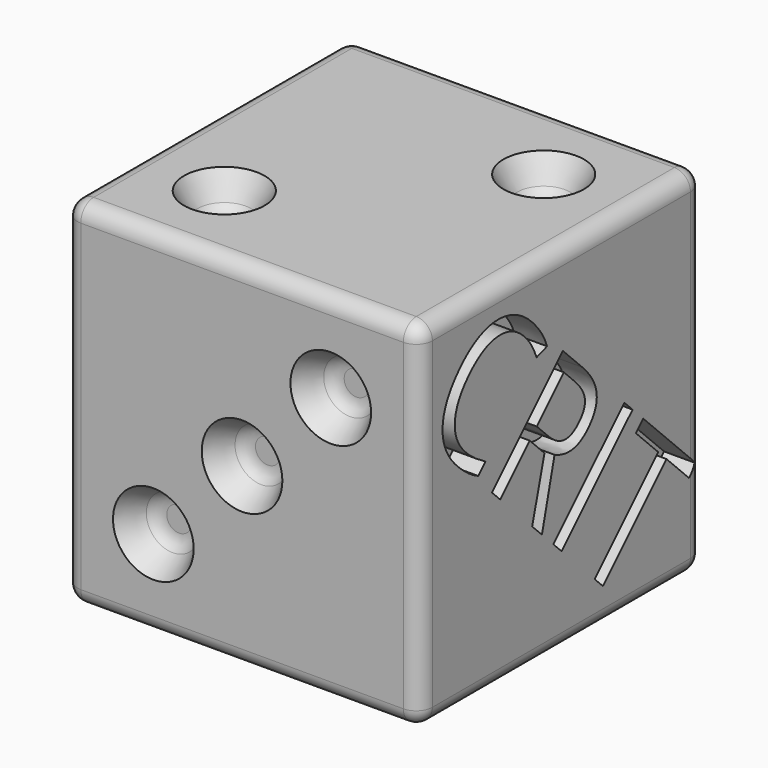
from build123d import *

# Parameters (mm, degrees)
F0_W          = 22
F0_H          = 22
F1_DEPTH      = 22
F2_R          = 2.5
F3_DEPTH      = 2
F3_TAPER      = 30
F4_R          = 2.5
F5_DEPTH      = 2
F5_TAPER      = 30
F6_R          = 2.5
F7_DEPTH      = 2
F7_TAPER      = 30
F8_R          = 2.5
F9_DEPTH      = 2
F9_TAPER      = 30
F10_R         = 2.5
F11_DEPTH     = 2
F11_TAPER     = 30
F12_TEXT_SIZE = 10.8916567981
F13_DEPTH     = 2
F14_T31_DEPTH = 20
F14_T33_DEPTH = 20
F14_T35_DEPTH = 20
F14_S39_W     = 1
F14_S39_H     = 1
F14_T40_DEPTH = 1
F14_S45_W     = 1
F14_S45_H     = 1
F14_T46_DEPTH = 1
F14_S51_W     = 1
F14_S51_H     = 1
F14_T52_DEPTH = 1
F14_S57_W     = 1
F14_S57_H     = 1
F14_T58_DEPTH = 1
F14_S63_W     = 1
F14_S63_H     = 1
F14_T64_DEPTH = 1
F14_S69_W     = 1
F14_S69_H     = 1
F14_T70_DEPTH = 1
F14_S75_W     = 1
F14_S75_H     = 1
F14_T76_DEPTH = 1
F14_S81_W     = 1
F14_S81_H     = 1
F14_T82_DEPTH = 1


# Not quite as in the source:
# - a fillet or chamfer that OpenCascade refuses, or shapes differently, is made with other operations: its cross-section is extruded or revolved along the edge and cut away or added
# - Text() gives the source's letters only with a copy of the font that has no kerning and outlines rounded to 1/6400 em; it was checked with that copy


with BuildPart() as f1:
    # F0 (on Top) → F1 (new body)
    with BuildSketch(Plane.XY):
        Rectangle(F0_W, F0_H)
    extrude(amount=F1_DEPTH)

    # F2 (on face) → F3 (cut)
    with BuildSketch(Plane(origin=(-11, 0, 0), x_dir=(0, -1, 0), z_dir=(-1, 0, 0))):
        with Locations((0, 11)):
            Circle(F2_R)
    extrude(amount=-F3_DEPTH, taper=F3_TAPER, mode=Mode.SUBTRACT)

    # F4 (on face) → F5 (cut)
    with BuildSketch(Plane.XY.offset(22)):
        with Locations((5.5, 5.5)):
            Circle(F4_R)
        with Locations((-5.5, -5.5)):
            Circle(F4_R)
    extrude(amount=-F5_DEPTH, taper=F5_TAPER, mode=Mode.SUBTRACT)

    # F6 (on face) → F7 (cut)
    with BuildSketch(Plane.XZ.offset(11)):
        with Locations((5.5, 16.5)):
            Circle(F6_R)
        with Locations((0, 11)):
            Circle(F6_R)
        with Locations((-5.5, 5.5)):
            Circle(F6_R)
    extrude(amount=-F7_DEPTH, taper=F7_TAPER, mode=Mode.SUBTRACT)

    # F8 (on face) → F9 (cut)
    with BuildSketch(Plane(origin=(0, 11, 0), x_dir=(-1, 0, 0), z_dir=(0, 1, 0))):
        with Locations((5.5, 16.5)):
            Circle(F8_R)
        with Locations((-5.5, 16.5)):
            Circle(F8_R)
        with Locations((5.5, 5.5)):
            Circle(F8_R)
        with Locations((-5.5, 5.5)):
            Circle(F8_R)
    extrude(amount=-F9_DEPTH, taper=F9_TAPER, mode=Mode.SUBTRACT)

    # F10 (on face) → F11 (cut)
    with BuildSketch(Plane(origin=(0, 0, 0), x_dir=(1, 0, 0), z_dir=(0, 0, -1))):
        Circle(F10_R)
        with Locations((5.5, -5.5)):
            Circle(F10_R)
        with Locations((-5.5, 5.5)):
            Circle(F10_R)
        with Locations((5.5, 5.5)):
            Circle(F10_R)
        with Locations((-5.5, -5.5)):
            Circle(F10_R)
    extrude(amount=-F11_DEPTH, taper=F11_TAPER, mode=Mode.SUBTRACT)

    # F12 (on face) → F13 (cut)
    with BuildSketch(Plane.YZ.offset(11)):
        with Locations(Location((-11, 16.4548736462), (0, 0, -45))):
            Text('CRIT', F12_TEXT_SIZE, font='Open Sans', text_align=(TextAlign.LEFT, TextAlign.BOTTOM))
    extrude(amount=-F13_DEPTH, mode=Mode.SUBTRACT)

    # F14: fillet of radius 1 on 27 edges, made by hand

    # F14_s1 → F14_t2 (revolve)
    with BuildSketch(Plane.XY.offset(16.5)):
        with BuildLine():
            ThreePointArc((-7.1339745962, 9.5), (-6.7679491924, 9.1339745962), (-6.2679491924, 9))
            Line((-6.2679491924, 9), (-6.8452994616, 9))
            Line((-6.8452994616, 9), (-7.1339745962, 9.5))
        make_face()
    revolve(axis=Axis((-5.5, 9, 16.5), (0, 1, 0)))

    # F14_s3 → F14_t4 (revolve)
    with BuildSketch(Plane.XY.offset(5.5)):
        with BuildLine():
            ThreePointArc((-7.1339745962, 9.5), (-6.7679491924, 9.1339745962), (-6.2679491924, 9))
            Line((-6.2679491924, 9), (-6.8452994616, 9))
            Line((-6.8452994616, 9), (-7.1339745962, 9.5))
        make_face()
    revolve(axis=Axis((-5.5, 9, 5.5), (0, 1, 0)))

    # F14_s5 → F14_t6 (revolve)
    with BuildSketch(Plane.XY.offset(5.5)):
        with BuildLine():
            ThreePointArc((3.8660254038, 9.5), (4.2320508076, 9.1339745962), (4.7320508076, 9))
            Line((4.7320508076, 9), (4.1547005384, 9))
            Line((4.1547005384, 9), (3.8660254038, 9.5))
        make_face()
    revolve(axis=Axis((5.5, 9, 5.5), (0, 1, 0)))

    # F14_s7 → F14_t8 (revolve)
    with BuildSketch(Plane.XY.offset(16.5)):
        with BuildLine():
            ThreePointArc((3.8660254038, 9.5), (4.2320508076, 9.1339745962), (4.7320508076, 9))
            Line((4.7320508076, 9), (4.1547005384, 9))
            Line((4.1547005384, 9), (3.8660254038, 9.5))
        make_face()
    revolve(axis=Axis((5.5, 9, 16.5), (0, 1, 0)))

    # F14_s9 → F14_t10 (revolve)
    with BuildSketch(Plane.XZ.offset(-5.5)):
        with BuildLine():
            ThreePointArc((7.1339745962, 20.5), (6.7679491924, 20.1339745962), (6.2679491924, 20))
            Line((6.2679491924, 20), (6.8452994616, 20))
            Line((6.8452994616, 20), (7.1339745962, 20.5))
        make_face()
    revolve(axis=Axis((5.5, 5.5, 20), (0, 0, 1)))

    # F14_s11 → F14_t12 (revolve)
    with BuildSketch(Plane.XZ.offset(5.5)):
        with BuildLine():
            ThreePointArc((-3.8660254038, 20.5), (-4.2320508076, 20.1339745962), (-4.7320508076, 20))
            Line((-4.7320508076, 20), (-4.1547005384, 20))
            Line((-4.1547005384, 20), (-3.8660254038, 20.5))
        make_face()
    revolve(axis=Axis((-5.5, -5.5, 20), (0, 0, 1)))

    # F14_s13 → F14_t14 (revolve)
    with BuildSketch(Plane.XZ.offset(-5.5)):
        with BuildLine():
            ThreePointArc((-3.8660254038, 1.5), (-4.2320508076, 1.8660254038), (-4.7320508076, 2))
            Line((-4.7320508076, 2), (-4.1547005384, 2))
            Line((-4.1547005384, 2), (-3.8660254038, 1.5))
        make_face()
    revolve(axis=Axis((-5.5, 5.5, 2), (0, 0, -1)))

    # F14_s15 → F14_t16 (revolve)
    with BuildSketch(Plane.XZ.offset(-5.5)):
        with BuildLine():
            ThreePointArc((7.1339745962, 1.5), (6.7679491924, 1.8660254038), (6.2679491924, 2))
            Line((6.2679491924, 2), (6.8452994616, 2))
            Line((6.8452994616, 2), (7.1339745962, 1.5))
        make_face()
    revolve(axis=Axis((5.5, 5.5, 2), (0, 0, -1)))

    # F14_s17 → F14_t18 (revolve)
    with BuildSketch(Plane.XZ):
        with BuildLine():
            ThreePointArc((1.6339745962, 1.5), (1.2679491924, 1.8660254038), (0.7679491924, 2))
            Line((0.7679491924, 2), (1.3452994616, 2))
            Line((1.3452994616, 2), (1.6339745962, 1.5))
        make_face()
    revolve(axis=Axis((0, 0, 2), (0, 0, -1)))

    # F14_s19 → F14_t20 (revolve)
    with BuildSketch(Plane.XZ.offset(5.5)):
        with BuildLine():
            ThreePointArc((7.1339745962, 1.5), (6.7679491924, 1.8660254038), (6.2679491924, 2))
            Line((6.2679491924, 2), (6.8452994616, 2))
            Line((6.8452994616, 2), (7.1339745962, 1.5))
        make_face()
    revolve(axis=Axis((5.5, -5.5, 2), (0, 0, -1)))

    # F14_s21 → F14_t22 (revolve)
    with BuildSketch(Plane.XZ.offset(5.5)):
        with BuildLine():
            ThreePointArc((-3.8660254038, 1.5), (-4.2320508076, 1.8660254038), (-4.7320508076, 2))
            Line((-4.7320508076, 2), (-4.1547005384, 2))
            Line((-4.1547005384, 2), (-3.8660254038, 1.5))
        make_face()
    revolve(axis=Axis((-5.5, -5.5, 2), (0, 0, -1)))

    # F14_s23 → F14_t24 (revolve)
    with BuildSketch(Plane.XY.offset(5.5)):
        with BuildLine():
            ThreePointArc((-3.8660254038, -9.5), (-4.2320508076, -9.1339745962), (-4.7320508076, -9))
            Line((-4.7320508076, -9), (-4.1547005384, -9))
            Line((-4.1547005384, -9), (-3.8660254038, -9.5))
        make_face()
    revolve(axis=Axis((-5.5, -9, 5.5), (0, -1, 0)))

    # F14_s25 → F14_t26 (revolve)
    with BuildSketch(Plane.XY.offset(11)):
        with BuildLine():
            ThreePointArc((1.6339745962, -9.5), (1.2679491924, -9.1339745962), (0.7679491924, -9))
            Line((0.7679491924, -9), (1.3452994616, -9))
            Line((1.3452994616, -9), (1.6339745962, -9.5))
        make_face()
    revolve(axis=Axis((0, -9, 11), (0, -1, 0)))

    # F14_s27 → F14_t28 (revolve)
    with BuildSketch(Plane.XY.offset(11)):
        with BuildLine():
            ThreePointArc((-9.5, -1.6339745962), (-9.1339745962, -1.2679491924), (-9, -0.7679491924))
            Line((-9, -0.7679491924), (-9, -1.3452994616))
            Line((-9, -1.3452994616), (-9.5, -1.6339745962))
        make_face()
    revolve(axis=Axis((-9, 0, 11), (-1, 0, 0)))

    # F14_s29 → F14_t30 (revolve)
    with BuildSketch(Plane.XY.offset(16.5)):
        with BuildLine():
            ThreePointArc((7.1339745962, -9.5), (6.7679491924, -9.1339745962), (6.2679491924, -9))
            Line((6.2679491924, -9), (6.8452994616, -9))
            Line((6.8452994616, -9), (7.1339745962, -9.5))
        make_face()
    revolve(axis=Axis((5.5, -9, 16.5), (0, -1, 0)))

    # F14_s32 → F14_t31 (cut)
    with BuildSketch(Plane.XY.offset(1)):
        with BuildLine():
            ThreePointArc((11, -10), (10.7071067812, -10.7071067812), (10, -11))
            Line((10, -11), (11, -11))
            Line((11, -11), (11, -10))
        make_face()
        with BuildLine():
            ThreePointArc((11, 10), (10.7071067812, 10.7071067812), (10, 11))
            Line((10, 11), (11, 11))
            Line((11, 11), (11, 10))
        make_face()
        with BuildLine():
            ThreePointArc((-10, -11), (-10.7071067812, -10.7071067812), (-11, -10))
            Line((-11, -10), (-11, -11))
            Line((-11, -11), (-10, -11))
        make_face()
        with BuildLine():
            ThreePointArc((-10, 11), (-10.7071067812, 10.7071067812), (-11, 10))
            Line((-11, 10), (-11, 11))
            Line((-11, 11), (-10, 11))
        make_face()
    extrude(amount=F14_T31_DEPTH, mode=Mode.SUBTRACT)

    # F14_s34 → F14_t33 (cut)
    with BuildSketch(Plane.XZ.offset(-10)):
        with BuildLine():
            ThreePointArc((11, 1), (10.7071067812, 0.2928932188), (10, 0))
            Line((10, 0), (11, 0))
            Line((11, 0), (11, 1))
        make_face()
        with BuildLine():
            ThreePointArc((11, 21), (10.7071067812, 21.7071067812), (10, 22))
            Line((10, 22), (11, 22))
            Line((11, 22), (11, 21))
        make_face()
        with BuildLine():
            ThreePointArc((-10, 0), (-10.7071067812, 0.2928932188), (-11, 1))
            Line((-11, 1), (-11, 0))
            Line((-11, 0), (-10, 0))
        make_face()
        with BuildLine():
            ThreePointArc((-10, 22), (-10.7071067812, 21.7071067812), (-11, 21))
            Line((-11, 21), (-11, 22))
            Line((-11, 22), (-10, 22))
        make_face()
    extrude(amount=F14_T33_DEPTH, mode=Mode.SUBTRACT)

    # F14_s36 → F14_t35 (cut)
    with BuildSketch(Plane.YZ.offset(-10)):
        with BuildLine():
            ThreePointArc((-11, 1), (-10.7071067812, 0.2928932188), (-10, 0))
            Line((-10, 0), (-11, 0))
            Line((-11, 0), (-11, 1))
        make_face()
        with BuildLine():
            ThreePointArc((10, 0), (10.7071067812, 0.2928932188), (11, 1))
            Line((11, 1), (11, 0))
            Line((11, 0), (10, 0))
        make_face()
        with BuildLine():
            ThreePointArc((-11, 21), (-10.7071067812, 21.7071067812), (-10, 22))
            Line((-10, 22), (-11, 22))
            Line((-11, 22), (-11, 21))
        make_face()
        with BuildLine():
            ThreePointArc((10, 22), (10.7071067812, 21.7071067812), (11, 21))
            Line((11, 21), (11, 22))
            Line((11, 22), (10, 22))
        make_face()
    extrude(amount=F14_T35_DEPTH, mode=Mode.SUBTRACT)


with BuildPart() as f14_tool38:
    # F14_s39 → F14_t40 (new body)
    with BuildSketch(Plane.YZ.offset(10)):
        with Locations((-10.5, 0.5)):
            Rectangle(F14_S39_W, F14_S39_H)
    extrude(amount=F14_T40_DEPTH)

    # F14_s41 → F14_t42 (revolve, cut)
    with BuildSketch(Plane(origin=(10, -10, 1), x_dir=(0, 0.7071067812, 0.7071067812), z_dir=(0, 0.7071067812, -0.7071067812))):
        with BuildLine():
            ThreePointArc((0, -1), (1, 0), (0, 1))
            Line((0, 1), (0, -1))
        make_face()
    revolve(axis=Axis((10, -10, 1), (1, 0, 0)), mode=Mode.SUBTRACT)


with BuildPart() as f1_1:
    add(f1.part)

    # F14_t37: cut F14_tool38
    add(f14_tool38.part, mode=Mode.SUBTRACT)


with BuildPart() as f14_tool44:
    # F14_s45 → F14_t46 (new body)
    with BuildSketch(Plane.YZ.offset(10)):
        with Locations((-10.5, 21.5)):
            Rectangle(F14_S45_W, F14_S45_H)
    extrude(amount=F14_T46_DEPTH)

    # F14_s47 → F14_t48 (revolve, cut)
    with BuildSketch(Plane(origin=(10, -10, 21), x_dir=(0, 0.7071067812, -0.7071067812), z_dir=(0, -0.7071067812, -0.7071067812))):
        with BuildLine():
            ThreePointArc((0, -1), (1, 0), (0, 1))
            Line((0, 1), (0, -1))
        make_face()
    revolve(axis=Axis((10, -10, 21), (1, 0, 0)), mode=Mode.SUBTRACT)


with BuildPart() as f1_2:
    add(f1_1.part)

    # F14_t43: cut F14_tool44
    add(f14_tool44.part, mode=Mode.SUBTRACT)


with BuildPart() as f14_tool50:
    # F14_s51 → F14_t52 (new body)
    with BuildSketch(Plane.YZ.offset(10)):
        with Locations((10.5, 0.5)):
            Rectangle(F14_S51_W, F14_S51_H)
    extrude(amount=F14_T52_DEPTH)

    # F14_s53 → F14_t54 (revolve, cut)
    with BuildSketch(Plane(origin=(10, 10, 1), x_dir=(0, -0.7071067812, 0.7071067812), z_dir=(0, 0.7071067812, 0.7071067812))):
        with BuildLine():
            ThreePointArc((0, -1), (1, 0), (0, 1))
            Line((0, 1), (0, -1))
        make_face()
    revolve(axis=Axis((10, 10, 1), (1, 0, 0)), mode=Mode.SUBTRACT)


with BuildPart() as f1_3:
    add(f1_2.part)

    # F14_t49: cut F14_tool50
    add(f14_tool50.part, mode=Mode.SUBTRACT)


with BuildPart() as f14_tool56:
    # F14_s57 → F14_t58 (new body)
    with BuildSketch(Plane.YZ.offset(10)):
        with Locations((10.5, 21.5)):
            Rectangle(F14_S57_W, F14_S57_H)
    extrude(amount=F14_T58_DEPTH)

    # F14_s59 → F14_t60 (revolve, cut)
    with BuildSketch(Plane(origin=(10, 10, 21), x_dir=(0, -0.7071067812, -0.7071067812), z_dir=(0, -0.7071067812, 0.7071067812))):
        with BuildLine():
            ThreePointArc((0, -1), (1, 0), (0, 1))
            Line((0, 1), (0, -1))
        make_face()
    revolve(axis=Axis((10, 10, 21), (1, 0, 0)), mode=Mode.SUBTRACT)


with BuildPart() as f1_4:
    add(f1_3.part)

    # F14_t55: cut F14_tool56
    add(f14_tool56.part, mode=Mode.SUBTRACT)


with BuildPart() as f14_tool62:
    # F14_s63 → F14_t64 (new body)
    with BuildSketch(Plane.XZ.offset(10)):
        with Locations((-10.5, 0.5)):
            Rectangle(F14_S63_W, F14_S63_H)
    extrude(amount=F14_T64_DEPTH)

    # F14_s65 → F14_t66 (revolve, cut)
    with BuildSketch(Plane(origin=(-10, -10, 1), x_dir=(0.7071067812, 0, 0.7071067812), z_dir=(0.7071067812, 0, -0.7071067812))):
        with BuildLine():
            ThreePointArc((0, -1), (1, 0), (0, 1))
            Line((0, 1), (0, -1))
        make_face()
    revolve(axis=Axis((-10, -10, 1), (0, -1, 0)), mode=Mode.SUBTRACT)


with BuildPart() as f1_5:
    add(f1_4.part)

    # F14_t61: cut F14_tool62
    add(f14_tool62.part, mode=Mode.SUBTRACT)


with BuildPart() as f14_tool68:
    # F14_s69 → F14_t70 (new body)
    with BuildSketch(Plane.XZ.offset(10)):
        with Locations((-10.5, 21.5)):
            Rectangle(F14_S69_W, F14_S69_H)
    extrude(amount=F14_T70_DEPTH)

    # F14_s71 → F14_t72 (revolve, cut)
    with BuildSketch(Plane(origin=(-10, -10, 21), x_dir=(0.7071067812, 0, -0.7071067812), z_dir=(-0.7071067812, 0, -0.7071067812))):
        with BuildLine():
            ThreePointArc((0, -1), (1, 0), (0, 1))
            Line((0, 1), (0, -1))
        make_face()
    revolve(axis=Axis((-10, -10, 21), (0, -1, 0)), mode=Mode.SUBTRACT)


with BuildPart() as f1_6:
    add(f1_5.part)

    # F14_t67: cut F14_tool68
    add(f14_tool68.part, mode=Mode.SUBTRACT)


with BuildPart() as f14_tool74:
    # F14_s75 → F14_t76 (new body)
    with BuildSketch(Plane.XY.offset(1)):
        with Locations((-10.5, 10.5)):
            Rectangle(F14_S75_W, F14_S75_H)
    extrude(amount=-F14_T76_DEPTH)

    # F14_s77 → F14_t78 (revolve, cut)
    with BuildSketch(Plane(origin=(-10, 10, 1), x_dir=(0.7071067812, -0.7071067812, 0), z_dir=(0.7071067812, 0.7071067812, 0))):
        with BuildLine():
            ThreePointArc((0, -1), (1, 0), (0, 1))
            Line((0, 1), (0, -1))
        make_face()
    revolve(axis=Axis((-10, 10, 1), (0, 0, -1)), mode=Mode.SUBTRACT)


with BuildPart() as f1_7:
    add(f1_6.part)

    # F14_t73: cut F14_tool74
    add(f14_tool74.part, mode=Mode.SUBTRACT)


with BuildPart() as f14_tool80:
    # F14_s81 → F14_t82 (new body)
    with BuildSketch(Plane.XY.offset(21)):
        with Locations((-10.5, 10.5)):
            Rectangle(F14_S81_W, F14_S81_H)
    extrude(amount=F14_T82_DEPTH)

    # F14_s83 → F14_t84 (revolve, cut)
    with BuildSketch(Plane(origin=(-10, 10, 21), x_dir=(0.7071067812, -0.7071067812, 0), z_dir=(-0.7071067812, -0.7071067812, 0))):
        with BuildLine():
            ThreePointArc((0, -1), (1, 0), (0, 1))
            Line((0, 1), (0, -1))
        make_face()
    revolve(axis=Axis((-10, 10, 21), (0, 0, 1)), mode=Mode.SUBTRACT)


with BuildPart() as f1_8:
    add(f1_7.part)

    # F14_t79: cut F14_tool80
    add(f14_tool80.part, mode=Mode.SUBTRACT)


solid = f1_8.part
